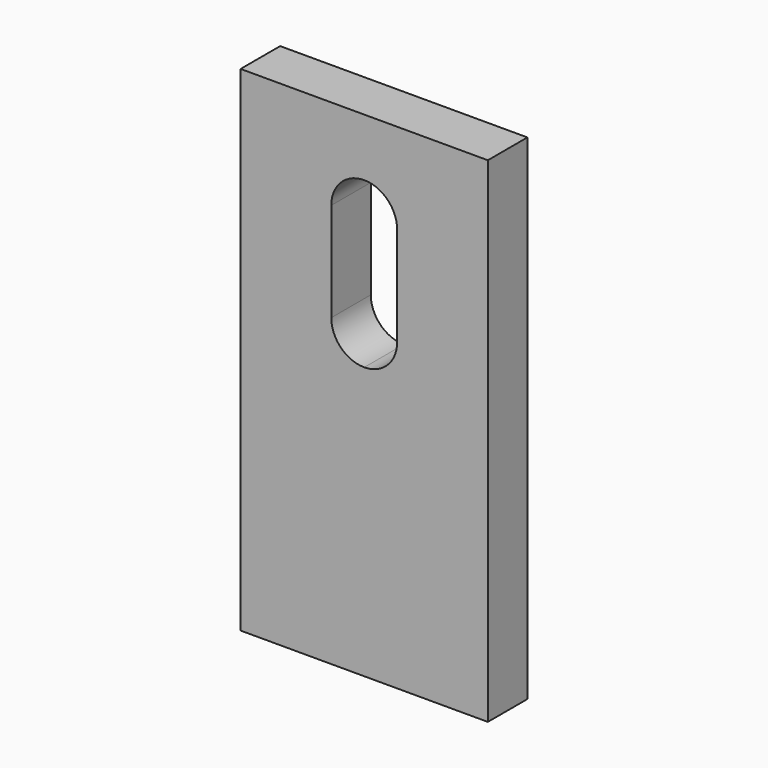
from build123d import *

# Parameters (mm, degrees)
F0_W     = 30
F0_H     = 60
F0_W_2   = 8
F0_H_2   = 20
F1_DEPTH = 6
F2_R     = 3.99999


# Not quite as in the source:
# - a fillet or chamfer is up to 0.001 mm smaller than in the source, because OpenCascade refuses the exact size


with BuildPart() as f1:
    # F0 (on Front) → F1 (new body)
    with BuildSketch(Plane.XZ):
        Rectangle(F0_W, F0_H)
        with Locations((0, 13)):
            Rectangle(F0_W_2, F0_H_2, mode=Mode.SUBTRACT)
    extrude(amount=F1_DEPTH)

    # F2 (radius 4 in the source; OpenCascade refuses exactly that, so slightly less here)
    f2_edges = [f1.edges().sort_by_distance(p)[0] for p in [
        (-4, -3, 23),
        (4, -3, 23),
        (-4, -3, 3),
        (4, -3, 3),
    ]]
    fillet(f2_edges, radius=F2_R)


solid = f1.part
